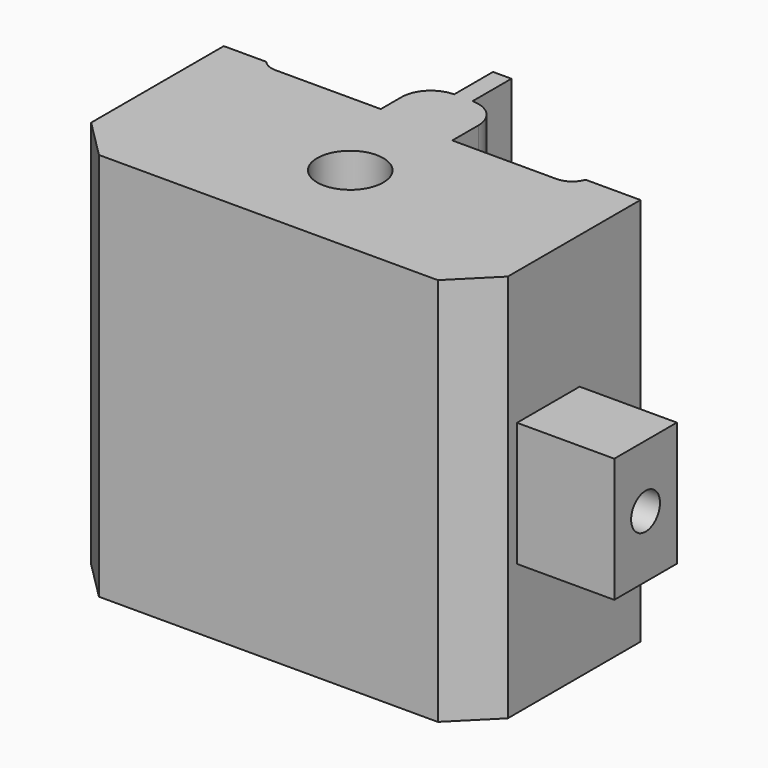
from build123d import *

# Parameters (mm, degrees)
F1_DEPTH     = 50.8
F2_DEPTH     = 12.7
F4_D         = 17.272
F5_DEPTH     = 76.2
F6_DEPTH     = 76.2
F7_W         = 20.4321481287
F7_H         = 32.4622914195
F8_DEPTH     = 25.4
F9_R         = 7.62
F10_SIZE     = 10.16
F12_D        = 9.4234
F13_DEPTH    = 12.7
F14_T1_DEPTH = 101.6


# Not quite as in the source:
# - a fillet or chamfer that OpenCascade refuses, or shapes differently, is made with other operations: its cross-section is extruded or revolved along the edge and cut away or added


with BuildPart() as f1:
    # F0 (on Top) → F1 (new body, symmetric)
    with BuildSketch(Plane.XY):
        Polygon((-44.3969555199, 12.5075299293), (-44.3969555199, 14.226121828), (-55.4723292589, 14.226121828), (-55.4723292589, -39.2411798239), (53.3718280494, -39.2411798239), (53.3718280494, 14.226121828), (39.0502288938, 14.226121828), (39.0502288938, 10.7889380306), (6.9698439911, 10.7889380306), (6.9698439911, 14.226121828), (-13.0803938955, 14.226121828), (-13.0803938955, 12.5075299293), align=None)
    extrude(amount=F1_DEPTH, both=True)

    # F2 (add): a face of the model
    f2_faces = [f1.faces().sort_by_distance(p)[0] for p in [
        (-3.0552749522, 14.226121828, 0),
    ]]
    extrude(f2_faces, amount=F2_DEPTH)

    # F4 (through all)
    with Locations(Plane(origin=(0, 0, -50.8), x_dir=(1, 0, 0), z_dir=(0, 0, -1))):
        with Locations((-1.0502506047, 12.507528998)):
            Hole(F4_D / 2)

    # F5 (add): a face of the model
    f5_faces = [f1.faces().sort_by_distance(p)[0] for p in [
        (-45.6707358145, 13.3668258786, 50.8),
    ]]
    extrude(f5_faces, amount=-F5_DEPTH)

    # F6 (add): a face of the model
    f6_faces = [f1.faces().sort_by_distance(p)[0] for p in [
        (-45.6707358145, 13.3668258786, 50.8),
    ]]
    extrude(f6_faces, amount=-F6_DEPTH)

    # F7 (on face) → F8 (join)
    with BuildSketch(Plane.YZ.offset(53.3718280494)):
        with Locations((-15.8492363989, -0.2864319831)):
            Rectangle(F7_W, F7_H)
    extrude(amount=F8_DEPTH)

    # F9
    f9_edges = [f1.edges().sort_by_distance(p)[0] for p in [
        (-13.080394, 26.926122, 0),
        (6.969844, 26.926122, 0),
    ]]
    fillet(f9_edges, radius=F9_R)

    # F10
    f10_edges = [f1.edges().sort_by_distance(p)[0] for p in [
        (53.371828, -39.24118, 0),
        (-55.472329, -39.24118, 0),
    ]]
    chamfer(f10_edges, length=F10_SIZE)

    # F12 (through all)
    with Locations(Plane.YZ.offset(78.7718280494)):
        with Locations((-15.8492363989, -0.2864319831)):
            Hole(F12_D / 2)

    # F13 (add): a face of the model
    f13_faces = [f1.faces().sort_by_distance(p)[0] for p in [
        (-3.0552749522, 26.926121828, 0),
    ]]
    extrude(f13_faces, amount=F13_DEPTH)

    # F14: fillet of radius 5.08 on 2 edges, made by hand

    # F14_s2 → F14_t1 (join)
    with BuildSketch(Plane.XY.offset(-50.8)):
        with BuildLine():
            ThreePointArc((-44.3969555199, 14.226121828), (-42.6774175907, 12.9570681189), (-40.5881058804, 12.5075299293))
            Line((-40.5881058804, 12.5075299293), (-44.3969555199, 12.5075299293))
            Line((-44.3969555199, 12.5075299293), (-44.3969555199, 14.226121828))
        make_face()
        with BuildLine():
            ThreePointArc((39.0502288938, 14.226121828), (37.1979300298, 11.7366319971), (34.2431970731, 10.7889380306))
            Line((34.2431970731, 10.7889380306), (39.0502288938, 10.7889380306))
            Line((39.0502288938, 10.7889380306), (39.0502288938, 14.226121828))
        make_face()
    extrude(amount=F14_T1_DEPTH)


solid = f1.part
